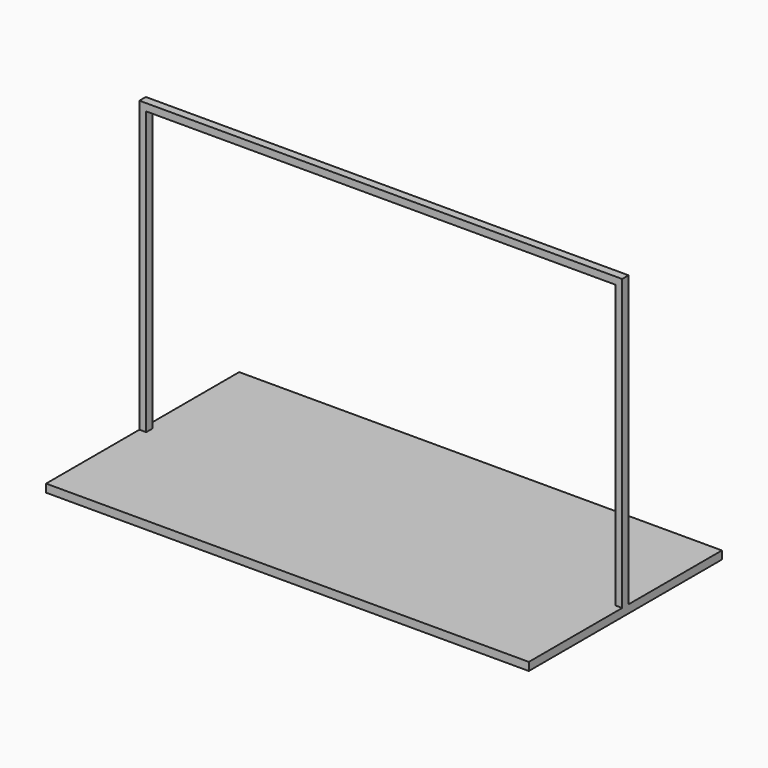
from build123d import *

# Parameters (mm, degrees)
F0_W     = 9144
F0_H     = 4572
F1_DEPTH = 152.4
F2_W     = 128.9591522217
F2_H     = 151.4181494713
F3_DEPTH = 5486.4
F4_W     = 151.4181494713
F4_H     = 136.9470108032
F5_DEPTH = 8886.0816955566


# Not quite as in the source:
# - the program builds the solid bodies; features that only make, move or delete a surface that nothing else refers to are left out


with BuildPart() as f1:
    # F0 (on Top) → F1 (new body)
    with BuildSketch(Plane.XY):
        Rectangle(F0_W, F0_H)
    extrude(amount=F1_DEPTH)

    # F2 (on face) → F3 (join)
    with BuildSketch(Plane.XY.offset(152.4)):
        with Locations((-4507.5204238892, 0)):
            Rectangle(F2_W, F2_H)
        with Locations((4507.5204238892, 0)):
            Rectangle(F2_W, F2_H)
    extrude(amount=F3_DEPTH)

    # F4 (on face) → F5 (join, through all)
    with BuildSketch(Plane.YZ.offset(-4443.0408477783)):
        with Locations((0, 5570.3264945984)):
            Rectangle(F4_W, F4_H)
    extrude(amount=F5_DEPTH)


solid = f1.part
